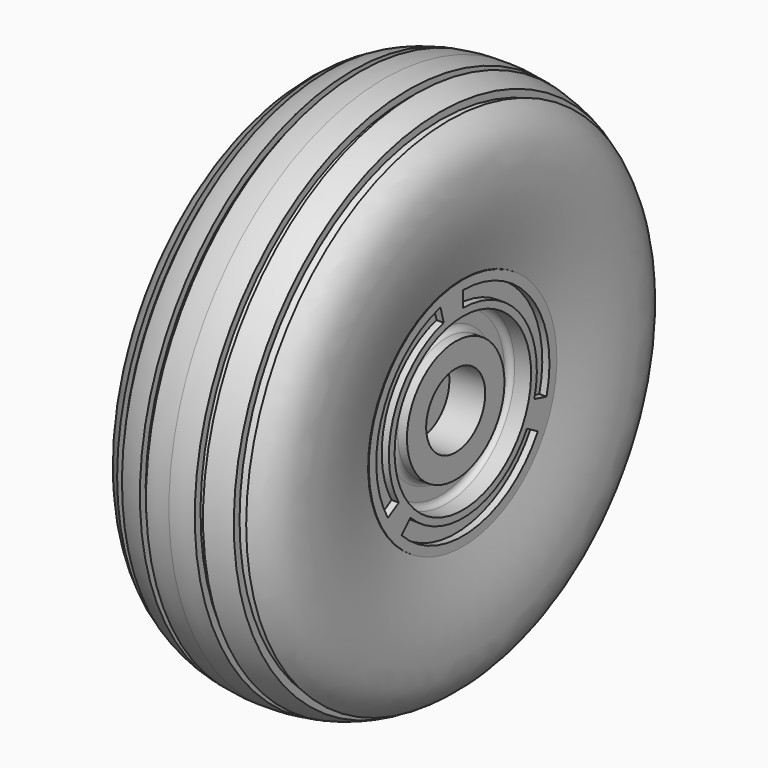
from build123d import *

# Parameters (mm, degrees)
F2_W            = 0.2
F2_H            = 0.22
F3_ANGLE        = 105
F3_COPIES_COUNT = 3


# Not quite as in the source:
# - a pattern or mirror of a feature is missing from the dataset's text; its kind, count and spacing are read off the source's solid


with BuildPart() as f1:
    # F0 (on Front) → F1 (revolve)
    with BuildSketch(Plane.XZ):
        with BuildLine():
            Line((1, 0.85), (0.87, 0.85))
            ThreePointArc((0.87, 0.85), (0.8134314575, 0.8734314575), (0.79, 0.93))
            Line((0.79, 0.93), (0.79, 1.11))
            ThreePointArc((0.79, 1.11), (0.8134314575, 1.1665685425), (0.87, 1.19))
            Line((0.87, 1.19), (1.1, 1.19))
            Line((1.1, 1.19), (1.1, 1.59))
            Line((1.1, 1.59), (1.1, 1.64))
            Line((1.1, 1.64), (1.0898001841, 1.64))
            add(Edge.make_bspline(
                [(1.0898001841, 1.64), (1.25, 2.278713374), (1.2631809244, 2.7012833679), (1.2262611325, 3.2585699441), (0.9876698715, 3.4728439225), (0.9, 3.5283316002)],
                knots=[0, 0, 0, 0, 0.3702653747, 0.6271589839, 0.7357428034, 0.7357428034, 0.7357428034, 0.7357428034], degree=3))
            Line((0.9, 3.5283316002), (0.9, 3.4283316002))
            Line((0.9, 3.4283316002), (0.78, 3.4941282527))
            Line((0.78, 3.4941282527), (0.78, 3.5941282527))
            add(Edge.make_bspline(
                [(0.78, 3.5941282527), (0.6808228027, 3.641181915), (0.5666603708, 3.6793418914), (0.44, 3.7061262113)],
                knots=[0.7816518304, 0.7816518304, 0.7816518304, 0.7816518304, 0.8878685464, 0.8878685464, 0.8878685464, 0.8878685464], degree=3))
            Line((0.44, 3.7061262113), (0.44, 3.6061262113))
            Line((0.44, 3.6061262113), (0.34, 3.6244667725))
            Line((0.34, 3.6244667725), (0.34, 3.7244667725))
            add(Edge.make_bspline(
                [(0.34, 3.7244667725), (0.2338131535, 3.7410670641), (0.120057055, 3.75), (0, 3.75)],
                knots=[0.9151424409, 0.9151424409, 0.9151424409, 0.9151424409, 1, 1, 1, 1], degree=3))
            Line((0, 3.75), (0, 0.515))
            Line((0, 0.515), (0, 0))
            Line((0, 0), (0.5, 0))
            Line((0.5, 0), (0.5, 0.515))
            Line((0.5, 0.515), (1, 0.515))
            Line((1, 0.515), (1, 0.85))
        make_face()
    revolve(axis=Axis((0.25, 0, 0), (1, 0, 0)))

    # F2 (on Front) → F3 (revolve, cut)
    with BuildSketch(Plane.XZ):
        with Locations((1.1, 1.4)):
            Rectangle(F2_W, F2_H)
    f3 = revolve(axis=Axis((1.36, 0, 0), (-1, 0, 0)), revolution_arc=F3_ANGLE, mode=Mode.SUBTRACT)

    # F3_copies: F3 ×3 about axis
    f3_copies_axis = Axis((0, 0, 0), (1, 0, 0))
    for i in range(1, F3_COPIES_COUNT):
        add(f3.rotate(f3_copies_axis, i * 360 / F3_COPIES_COUNT), mode=Mode.SUBTRACT)

    # F4: F1 across face


with BuildPart() as f1_1:
    add(f1.part)
    add(f1.part.mirror(Plane(origin=(0, 0, 0), x_dir=(0, -1, 0), z_dir=(-1, 0, 0))))


solid = f1_1.part
